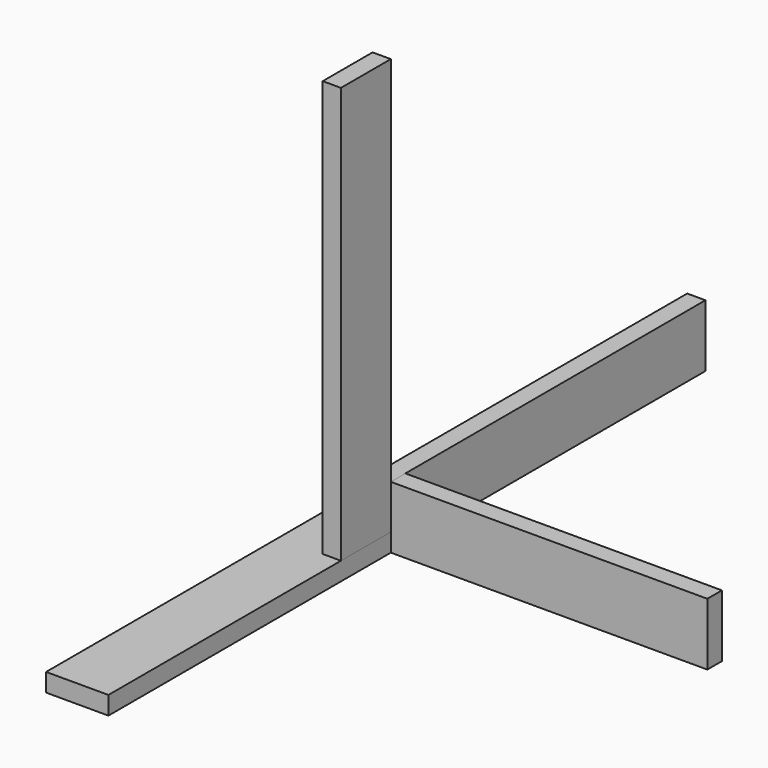
from build123d import *

# Parameters (mm, degrees)
F0_W     = 19
F0_H     = 65
F1_DEPTH = 330
F3_W     = 19
F3_H     = 65
F4_DEPTH = 410
F2_W     = 19
F2_H     = 65
F5_DEPTH = 453
F6_W     = 65
F6_H     = 19
F7_DEPTH = 368


# Not quite as in the source:
# - a feature names something its author has since deleted; it is built from what else it names


with BuildPart() as f1:
    # F0 (on Right) → F1 (new body)
    with BuildSketch(Plane.YZ):
        with Locations((9.5, 32.5)):
            Rectangle(F0_W, F0_H)
    extrude(amount=F1_DEPTH)


with BuildPart() as f4:
    # F3 (on Front) → F4 (new body)
    with BuildSketch(Plane.XZ):
        with Locations((-9.5, 32.5)):
            Rectangle(F3_W, F3_H)
    extrude(amount=-F4_DEPTH)


with BuildPart() as f5:
    # F2 (on Top) → F5 (new body)
    with BuildSketch(Plane.XY):
        with Locations((-9.5, -32.5)):
            Rectangle(F2_W, F2_H)
    extrude(amount=F5_DEPTH)


with BuildPart() as f7:
    # F6 (on Front) → F7 (new body)
    with BuildSketch(Plane.XZ):
        with Locations((-32.5, 9.5)):
            Rectangle(F6_W, F6_H)
    extrude(amount=F7_DEPTH)


solid = Compound([f1.part, f4.part, f5.part, f7.part])
